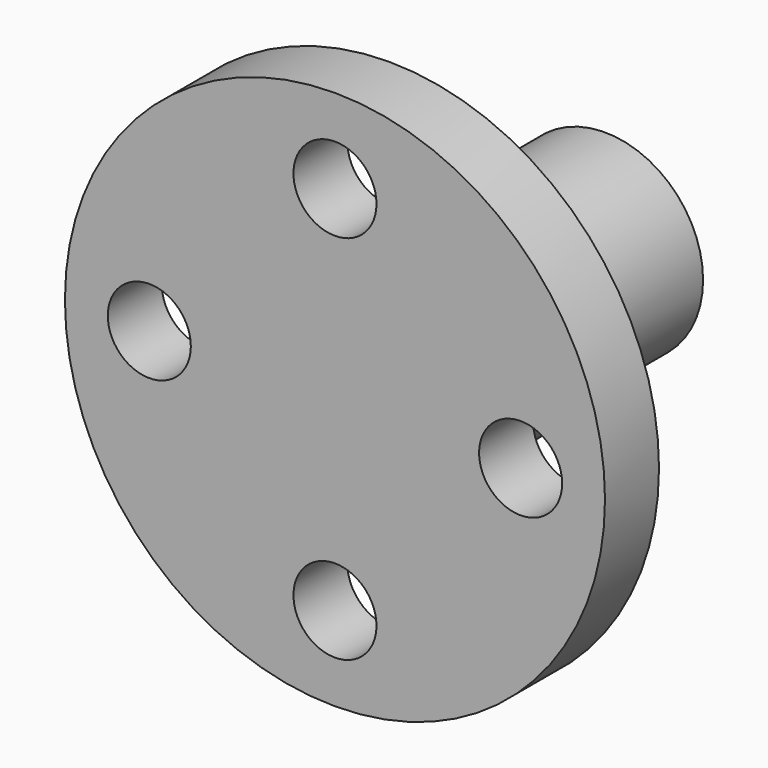
from build123d import *

# Parameters (mm, degrees)
F0_R     = 4.6125
F1_DEPTH = 6.35
F2_R     = 4.9625
F3_DEPTH = 6.35
F4_R     = 12.7
F4_R_2   = 1.9526
F5_DEPTH = 3.175


# Not quite as in the source:
# - a length typed as a fraction of an inch, garbled in the dataset ("3 / 203.2 mm" for 3/8 in), is restored


with BuildPart() as f1:
    # F0 (on Front) → F1 (new body)
    with BuildSketch(Plane.XZ):
        Circle(F0_R)
    extrude(amount=F1_DEPTH)

    # F2 (on face) → F3 (join)
    with BuildSketch(Plane.XZ.offset(6.35)):
        Circle(F2_R)
    extrude(amount=F3_DEPTH)

    # F4 (on face) → F5 (join)
    with BuildSketch(Plane.XZ.offset(12.7)):
        Circle(F4_R)
        with Locations((0, -8.73125)):
            Circle(F4_R_2, mode=Mode.SUBTRACT)
        with Locations((-8.73125, 0)):
            Circle(F4_R_2, mode=Mode.SUBTRACT)
        with Locations((8.73125, 0)):
            Circle(F4_R_2, mode=Mode.SUBTRACT)
        with Locations((0, 8.73125)):
            Circle(F4_R_2, mode=Mode.SUBTRACT)
    extrude(amount=F5_DEPTH)


solid = f1.part
